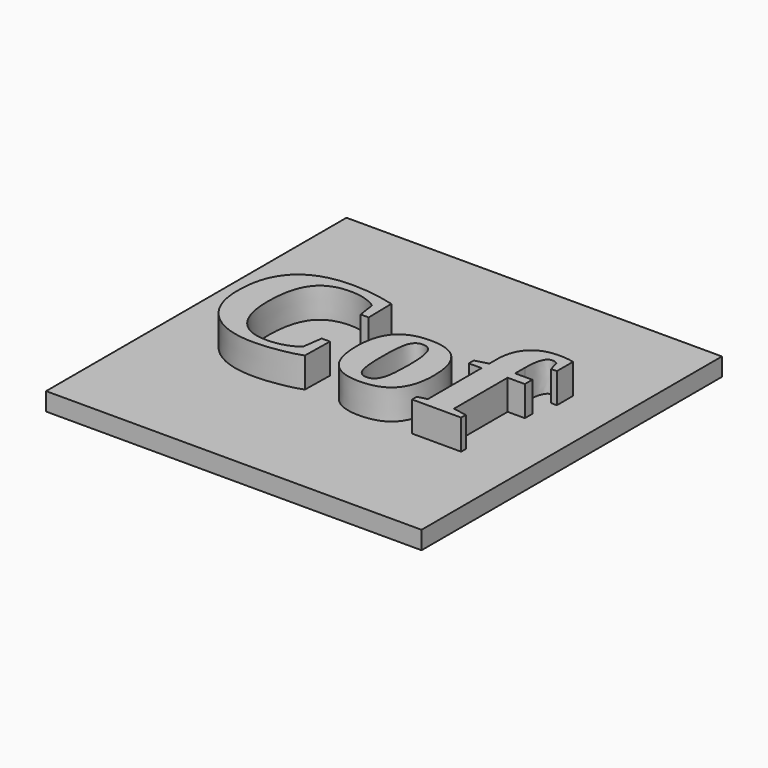
from build123d import *

# Parameters (mm, degrees)
F0_W         = 25
F0_H         = 25
F1_DEPTH     = 1.2
F2_TEXT_SIZE = 12.2887864823
F3_DEPTH     = 2


# Not quite as in the source:
# - Text() gives the source's letters only with a copy of the font that has no kerning and outlines rounded to 1/6400 em; it was checked with that copy


with BuildPart() as f1:
    # F0 (on Top) → F1 (new body)
    with BuildSketch(Plane.XY):
        Rectangle(F0_W, F0_H)
    extrude(amount=F1_DEPTH)

    # F2 (on face) → F3 (join)
    with BuildSketch(Plane.XY.offset(1.2)):
        with Locations((-10, -4.3479262673)):
            Text('Cof', F2_TEXT_SIZE, font='Tinos', font_style=FontStyle.BOLD, text_align=(TextAlign.LEFT, TextAlign.BOTTOM))
    extrude(amount=F3_DEPTH)


solid = f1.part
